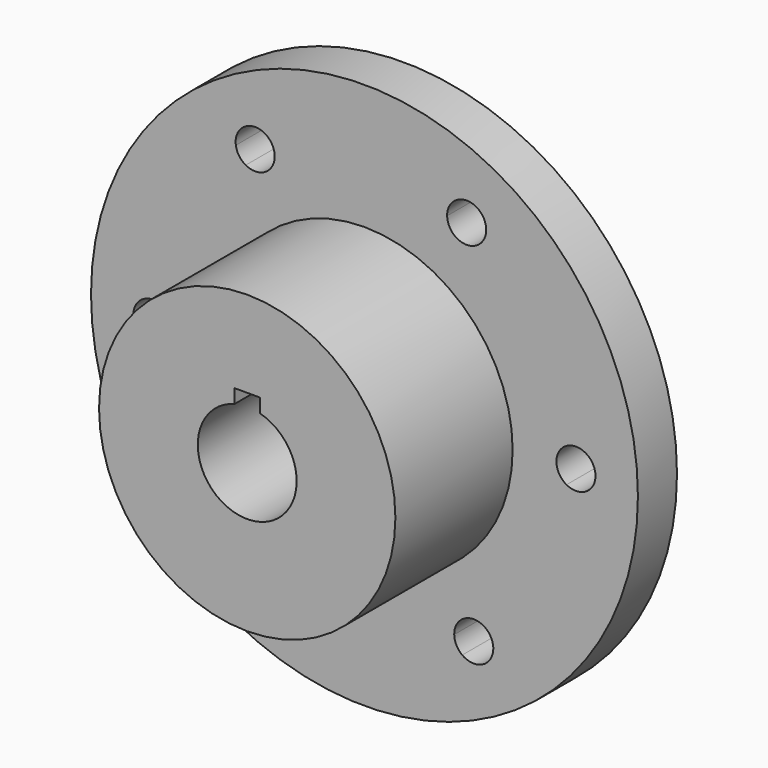
from build123d import *

# Parameters (mm, degrees)
F0_R     = 19.2609735147
F0_R_2   = 12.2005703348
F1_DEPTH = 25.4
F0_R_3   = 35.5458123626
F0_R_4   = 2.54
F2_DEPTH = 6.35
F3_DEPTH = 6.35


# Not quite as in the source:
# - a feature names something its author has since deleted; it is built from what else it names


with BuildPart() as f1:
    # F0 (on Front) → F1 (new body)
    with BuildSketch(Plane.XZ):
        Circle(F0_R)
        Circle(F0_R_2, mode=Mode.SUBTRACT)
        Circle(F0_R_2)
        with BuildLine():
            ThreePointArc((1.651, 6.2104947822), (0, -6.4262), (-1.651, 6.2104947822))
            Line((-1.651, 6.2104947822), (-1.651, 8.0264))
            Line((-1.651, 8.0264), (1.651, 8.0264))
            Line((1.651, 8.0264), (1.651, 6.2104947822))
        make_face(mode=Mode.SUBTRACT)
    extrude(amount=F1_DEPTH)


with BuildPart() as f2:
    # F0 (on Front) → F2 (new body)
    with BuildSketch(Plane.XZ):
        Circle(F0_R_3)
        with BuildLine():
            ThreePointArc((-15.8102357857, -23.8026693755), (-15.4266913627, -22.7088700736), (-14.5971077055, -21.899367638))
            ThreePointArc((-14.5971077055, -21.899367638), (-12.0575833253, -21.8502156048), (-10.7452542258, -24.024932215))
            ThreePointArc((-10.7452542258, -24.024932215), (-10.7448975137, -24.0495070811), (-10.744778606, -24.0740842482))
            ThreePointArc((-10.744778606, -24.0740842482), (-10.9984346498, -25.1805341179), (-11.7087402706, -26.0659936752))
            ThreePointArc((-11.7087402706, -26.0659936752), (-14.5119738867, -26.2979528916), (-15.8102357857, -23.8026693755))
        make_face(mode=Mode.SUBTRACT)
        with Locations((-27.4911578348, -0.5320863677)):
            Circle(F0_R_4, mode=Mode.SUBTRACT)
        with BuildLine():
            ThreePointArc((12.7085984642, -25.593400518), (11.9531126936, -24.7143416532), (11.6668548486, -23.5911499138))
            ThreePointArc((11.6668548486, -23.5911499138), (12.8940501293, -21.3672812704), (15.4335745095, -21.3181292371))
            ThreePointArc((15.4335745095, -21.3181292371), (16.2938606715, -22.0949245492), (16.7194425623, -23.1730633582))
            ThreePointArc((16.7194425623, -23.1730633582), (16.7396361115, -23.3570395976), (16.7463792288, -23.5419978805))
            ThreePointArc((16.7463792288, -23.5419978805), (15.3568653995, -25.8065025882), (12.7085984642, -25.593400518))
        make_face(mode=Mode.SUBTRACT)
        with BuildLine():
            ThreePointArc((-12.7085984642, 25.593400518), (-11.9531126936, 24.7143416532), (-11.6668548486, 23.5911499138))
            ThreePointArc((-11.6668548486, 23.5911499138), (-11.6664981365, 23.5665750477), (-11.6663792288, 23.5419978805))
            ThreePointArc((-11.6663792288, 23.5419978805), (-12.9151542316, 21.3546849156), (-15.4335745095, 21.3181292371))
            ThreePointArc((-15.4335745095, 21.3181292371), (-16.2938606715, 22.0949245492), (-16.7194425623, 23.1730633582))
            ThreePointArc((-16.7194425623, 23.1730633582), (-15.5187083283, 25.7167144907), (-12.7085984642, 25.593400518))
        make_face(mode=Mode.SUBTRACT)
        Circle(F0_R, mode=Mode.SUBTRACT)
        with BuildLine():
            ThreePointArc((28.5188342499, -1.7907311425), (27.3798040563, -2.0054715796), (26.2639625541, -1.6917822757))
            ThreePointArc((26.2639625541, -1.6917822757), (24.9516334546, 0.4829343345), (26.1788287353, 2.7068029779))
            ThreePointArc((26.1788287353, 2.7068029779), (27.2816962901, 3.0634349927), (28.4281828329, 2.892930317))
            ThreePointArc((28.4281828329, 2.892930317), (29.592543508, 1.9588933807), (30.0311578348, 0.5320863677))
            ThreePointArc((30.0311578348, 0.5320863677), (29.6197604391, -0.8537891508), (28.5188342499, -1.7907311425))
        make_face(mode=Mode.SUBTRACT)
        with BuildLine():
            ThreePointArc((15.8102357857, 23.8026693755), (15.4266913627, 22.7088700736), (14.5971077055, 21.899367638))
            ThreePointArc((14.5971077055, 21.899367638), (12.0575833253, 21.8502156048), (10.7452542258, 24.024932215))
            ThreePointArc((10.7452542258, 24.024932215), (10.9878356185, 25.1583595419), (11.7087402706, 26.0659936752))
            ThreePointArc((11.7087402706, 26.0659936752), (14.3912284756, 26.3604282044), (15.824778606, 24.0740842482))
            ThreePointArc((15.824778606, 24.0740842482), (15.8211402951, 23.9381821449), (15.8102357857, 23.8026693755))
        make_face(mode=Mode.SUBTRACT)
    extrude(amount=F2_DEPTH)


with BuildPart() as f3:
    # F0 (on Front) → F3 (new body)
    with BuildSketch(Plane.XZ):
        Circle(F0_R_3)
        with BuildLine():
            ThreePointArc((-15.8102357857, -23.8026693755), (-15.4266913627, -22.7088700736), (-14.5971077055, -21.899367638))
            ThreePointArc((-14.5971077055, -21.899367638), (-12.0575833253, -21.8502156048), (-10.7452542258, -24.024932215))
            ThreePointArc((-10.7452542258, -24.024932215), (-10.7448975137, -24.0495070811), (-10.744778606, -24.0740842482))
            ThreePointArc((-10.744778606, -24.0740842482), (-10.9984346498, -25.1805341179), (-11.7087402706, -26.0659936752))
            ThreePointArc((-11.7087402706, -26.0659936752), (-14.5119738867, -26.2979528916), (-15.8102357857, -23.8026693755))
        make_face(mode=Mode.SUBTRACT)
        with Locations((-27.4911578348, -0.5320863677)):
            Circle(F0_R_4, mode=Mode.SUBTRACT)
        with BuildLine():
            ThreePointArc((12.7085984642, -25.593400518), (11.9531126936, -24.7143416532), (11.6668548486, -23.5911499138))
            ThreePointArc((11.6668548486, -23.5911499138), (12.8940501293, -21.3672812704), (15.4335745095, -21.3181292371))
            ThreePointArc((15.4335745095, -21.3181292371), (16.2938606715, -22.0949245492), (16.7194425623, -23.1730633582))
            ThreePointArc((16.7194425623, -23.1730633582), (16.7396361115, -23.3570395976), (16.7463792288, -23.5419978805))
            ThreePointArc((16.7463792288, -23.5419978805), (15.3568653995, -25.8065025882), (12.7085984642, -25.593400518))
        make_face(mode=Mode.SUBTRACT)
        with BuildLine():
            ThreePointArc((-12.7085984642, 25.593400518), (-11.9531126936, 24.7143416532), (-11.6668548486, 23.5911499138))
            ThreePointArc((-11.6668548486, 23.5911499138), (-11.6664981365, 23.5665750477), (-11.6663792288, 23.5419978805))
            ThreePointArc((-11.6663792288, 23.5419978805), (-12.9151542316, 21.3546849156), (-15.4335745095, 21.3181292371))
            ThreePointArc((-15.4335745095, 21.3181292371), (-16.2938606715, 22.0949245492), (-16.7194425623, 23.1730633582))
            ThreePointArc((-16.7194425623, 23.1730633582), (-15.5187083283, 25.7167144907), (-12.7085984642, 25.593400518))
        make_face(mode=Mode.SUBTRACT)
        Circle(F0_R, mode=Mode.SUBTRACT)
        with BuildLine():
            ThreePointArc((28.5188342499, -1.7907311425), (27.3798040563, -2.0054715796), (26.2639625541, -1.6917822757))
            ThreePointArc((26.2639625541, -1.6917822757), (24.9516334546, 0.4829343345), (26.1788287353, 2.7068029779))
            ThreePointArc((26.1788287353, 2.7068029779), (27.2816962901, 3.0634349927), (28.4281828329, 2.892930317))
            ThreePointArc((28.4281828329, 2.892930317), (29.592543508, 1.9588933807), (30.0311578348, 0.5320863677))
            ThreePointArc((30.0311578348, 0.5320863677), (29.6197604391, -0.8537891508), (28.5188342499, -1.7907311425))
        make_face(mode=Mode.SUBTRACT)
        with BuildLine():
            ThreePointArc((15.8102357857, 23.8026693755), (15.4266913627, 22.7088700736), (14.5971077055, 21.899367638))
            ThreePointArc((14.5971077055, 21.899367638), (12.0575833253, 21.8502156048), (10.7452542258, 24.024932215))
            ThreePointArc((10.7452542258, 24.024932215), (10.9878356185, 25.1583595419), (11.7087402706, 26.0659936752))
            ThreePointArc((11.7087402706, 26.0659936752), (14.3912284756, 26.3604282044), (15.824778606, 24.0740842482))
            ThreePointArc((15.824778606, 24.0740842482), (15.8211402951, 23.9381821449), (15.8102357857, 23.8026693755))
        make_face(mode=Mode.SUBTRACT)
    extrude(amount=F3_DEPTH)


solid = Compound([f1.part, f2.part, f3.part])
